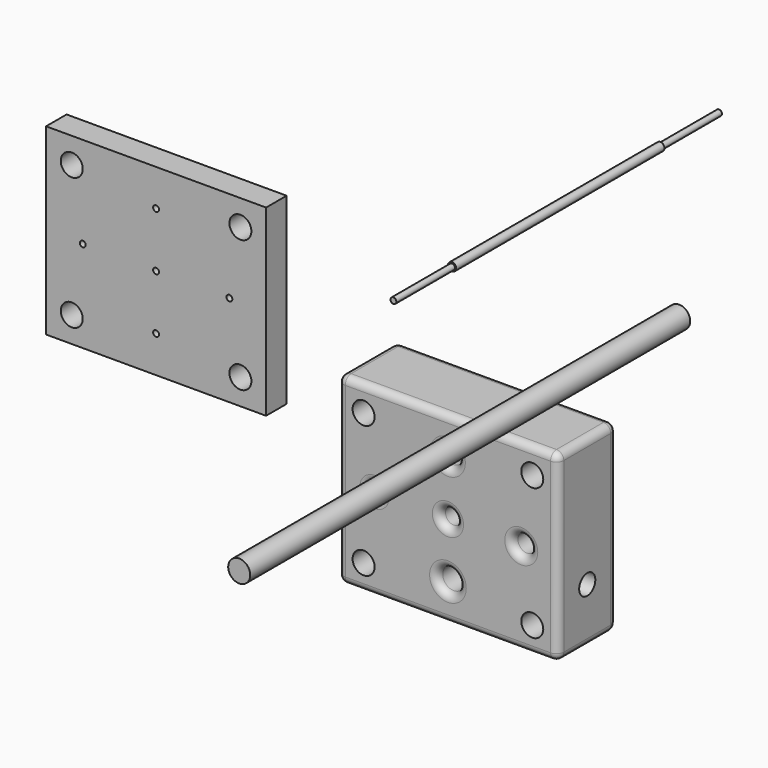
from build123d import *

# Parameters (mm, degrees)
F0_W         = 60
F0_H         = 50
F0_R         = 3
F0_R_2       = 2
F0_R_3       = 2.25
F0_R_4       = 2.5
F0_R_5       = 2.75
F1_DEPTH     = 20
F3_D         = 5.5
F3_DEPTH     = 7
F3_TIP       = 1.6523667023
F4_R         = 2
F5_R         = 2
F6_R         = 2
F7_T1_DEPTH  = 16
F7_S5_W      = 2
F7_S5_H      = 2
F7_T6_DEPTH  = 2
F7_S11_W     = 2
F7_S11_H     = 2
F7_T12_DEPTH = 2
F10_W        = 60
F10_H        = 50
F10_R        = 3
F10_R_2      = 0.8
F11_DEPTH    = 7
F12_R        = 3
F13_DEPTH    = 150


# Not quite as in the source:
# - a fillet or chamfer that OpenCascade refuses, or shapes differently, is made with other operations: its cross-section is extruded or revolved along the edge and cut away or added


with BuildPart() as f1:
    # F0 (on Front) → F1 (new body)
    with BuildSketch(Plane.XZ):
        Rectangle(F0_W, F0_H)
        with Locations((-23, -18)):
            Circle(F0_R, mode=Mode.SUBTRACT)
        with Locations((0, -15)):
            Circle(F0_R, mode=Mode.SUBTRACT)
        with Locations((23, -18)):
            Circle(F0_R, mode=Mode.SUBTRACT)
        with Locations((-20, 0)):
            Circle(F0_R_2, mode=Mode.SUBTRACT)
        with Locations((-23, 18)):
            Circle(F0_R, mode=Mode.SUBTRACT)
        Circle(F0_R_3, mode=Mode.SUBTRACT)
        with Locations((20, 0)):
            Circle(F0_R_4, mode=Mode.SUBTRACT)
        with Locations((0, 15)):
            Circle(F0_R_5, mode=Mode.SUBTRACT)
        with Locations((23, 18)):
            Circle(F0_R, mode=Mode.SUBTRACT)
    extrude(amount=F1_DEPTH)

    # F3
    with Locations(Plane.YZ.offset(30)):
        with Locations((-10, -10)):
            Hole(F3_D / 2, depth=F3_DEPTH)
            with Locations((0, 0, -(F3_DEPTH + F3_TIP / 2))):  # 118° drill point
                Cone(0, F3_D / 2, F3_TIP, mode=Mode.SUBTRACT)

    # F4
    f4_edges = [f1.edges().sort_by_distance(p)[0] for p in [
        (0, -20, 25),
        (0, 0, 25),
        (-30, -10, 25),
        (-30, -20, 0),
        (-30, 0, 0),
        (30, -10, 25),
        (30, 0, 0),
        (30, -20, 0),
        (30, -10, -25),
        (0, -20, -25),
        (0, 0, -25),
    ]]
    fillet(f4_edges, radius=F4_R)

    # F5
    f5_edges = [f1.edges().sort_by_distance(p)[0] for p in [
        (-3, -20, -15),
        (-22, -20, 0),
        (-2.75, -20, 15),
        (-2.25, -20, 0),
        (17.5, -20, 0),
        (-3, 0, -15),
        (17.5, 0, 0),
        (-22, 0, 0),
        (-2.75, 0, 15),
    ]]
    fillet(f5_edges, radius=F5_R)

    # F6
    f6_edges = [f1.edges().sort_by_distance(p)[0] for p in [
        (-2.25, 0, 0),
    ]]
    fillet(f6_edges, radius=F6_R)

    # F7: fillet of radius 2 on 1 edges, made by hand

    # F7_s2 → F7_t1 (cut)
    with BuildSketch(Plane.XZ.offset(2)):
        with BuildLine():
            ThreePointArc((-30, -23), (-29.4142135624, -24.4142135624), (-28, -25))
            Line((-28, -25), (-30, -25))
            Line((-30, -25), (-30, -23))
        make_face()
    extrude(amount=F7_T1_DEPTH, mode=Mode.SUBTRACT)


with BuildPart() as f7_tool4:
    # F7_s5 → F7_t6 (new body)
    with BuildSketch(Plane.YZ.offset(-28)):
        with Locations((-1, -24)):
            Rectangle(F7_S5_W, F7_S5_H)
    extrude(amount=-F7_T6_DEPTH)

    # F7_s7 → F7_t8 (revolve, cut)
    with BuildSketch(Plane(origin=(-28, -2, -23), x_dir=(0, -0.7071067812, 0.7071067812), z_dir=(0, -0.7071067812, -0.7071067812))):
        with BuildLine():
            ThreePointArc((0, -2), (2, 0), (0, 2))
            Line((0, 2), (0, -2))
        make_face()
    revolve(axis=Axis((-28, -2, -23), (-1, 0, 0)), mode=Mode.SUBTRACT)


with BuildPart() as f1_1:
    add(f1.part)

    # F7_t3: cut F7_tool4
    add(f7_tool4.part, mode=Mode.SUBTRACT)


with BuildPart() as f7_tool10:
    # F7_s11 → F7_t12 (new body)
    with BuildSketch(Plane.YZ.offset(-28)):
        with Locations((-19, -24)):
            Rectangle(F7_S11_W, F7_S11_H)
    extrude(amount=-F7_T12_DEPTH)

    # F7_s13 → F7_t14 (revolve, cut)
    with BuildSketch(Plane(origin=(-28, -18, -23), x_dir=(0, 0.7071067812, 0.7071067812), z_dir=(0, -0.7071067812, 0.7071067812))):
        with BuildLine():
            ThreePointArc((0, -2), (2, 0), (0, 2))
            Line((0, 2), (0, -2))
        make_face()
    revolve(axis=Axis((-28, -18, -23), (-1, 0, 0)), mode=Mode.SUBTRACT)


with BuildPart() as f1_2:
    add(f1_1.part)

    # F7_t9: cut F7_tool10
    add(f7_tool10.part, mode=Mode.SUBTRACT)


with BuildPart() as f9:
    # F8 (on Right) → F9 (revolve)
    with BuildSketch(Plane.YZ):
        Polygon((72.4104943052, 59.2), (72.4104943052, 60), (-38.5895056948, 60), (-38.5895056948, 59.2), (-18.5895056948, 59.2), (-18.5895056948, 58.875), (52.4104943052, 58.875), (52.4104943052, 59.2), align=None)
    revolve(axis=Axis((0, 16.9104943052, 60), (0, -1, 0)))


with BuildPart() as f11:
    # F10 (on Front) → F11 (new body)
    with BuildSketch(Plane.XZ):
        with Locations((-90, 25)):
            Rectangle(F10_W, F10_H)
        with Locations((-113, 7)):
            Circle(F10_R, mode=Mode.SUBTRACT)
        with Locations((-90, 10)):
            Circle(F10_R_2, mode=Mode.SUBTRACT)
        with Locations((-67, 7)):
            Circle(F10_R, mode=Mode.SUBTRACT)
        with Locations((-110, 25)):
            Circle(F10_R_2, mode=Mode.SUBTRACT)
        with Locations((-113, 43)):
            Circle(F10_R, mode=Mode.SUBTRACT)
        with Locations((-90, 25)):
            Circle(F10_R_2, mode=Mode.SUBTRACT)
        with Locations((-70, 25)):
            Circle(F10_R_2, mode=Mode.SUBTRACT)
        with Locations((-90, 40)):
            Circle(F10_R_2, mode=Mode.SUBTRACT)
        with Locations((-67, 43)):
            Circle(F10_R, mode=Mode.SUBTRACT)
    extrude(amount=F11_DEPTH)


with BuildPart() as f13:
    # F12 (on Front) → F13 (new body)
    with BuildSketch(Plane.XZ):
        with Locations((47.0741167665, 55.6864440441)):
            Circle(F12_R)
    extrude(amount=F13_DEPTH)


solid = Compound([f1_2.part, f9.part, f11.part, f13.part])
